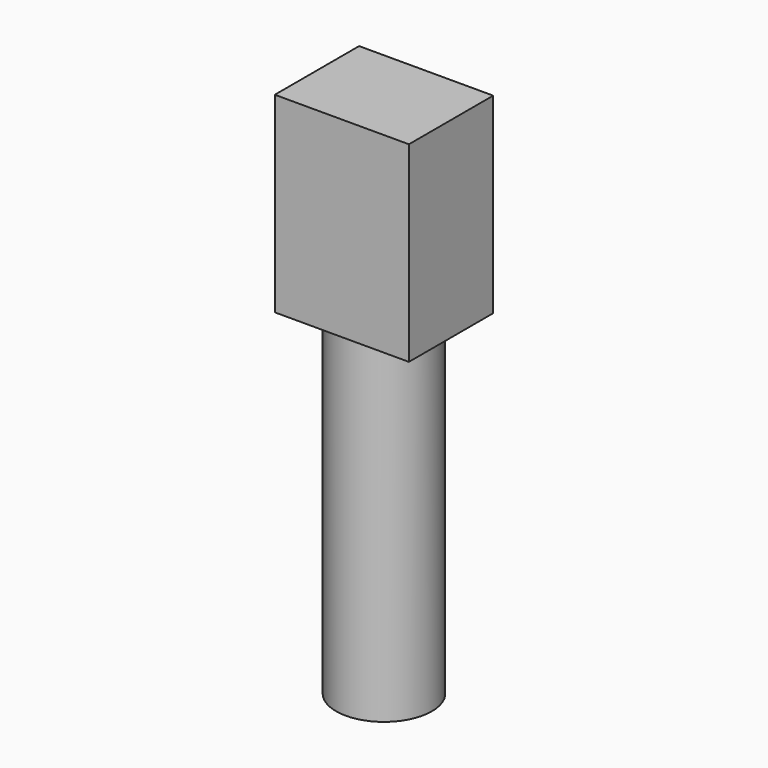
from build123d import *

# Parameters (mm, degrees)
F0_R     = 50
F1_DEPTH = 350
F2_W     = 140
F2_H     = 110
F2_R     = 50
F3_DEPTH = 200


# Not quite as in the source:
# - a feature names something its author has since deleted; it is built from what else it names


with BuildPart() as f1:
    # F0 (on Top) → F1 (new body)
    with BuildSketch(Plane.XY):
        Circle(F0_R)
    extrude(amount=F1_DEPTH)

    # F2 (on face) → F3 (join)
    with BuildSketch(Plane.XY.offset(350)):
        Rectangle(F2_W, F2_H)
        Circle(F2_R, mode=Mode.SUBTRACT)
        Circle(F2_R)
    extrude(amount=F3_DEPTH)


solid = f1.part
